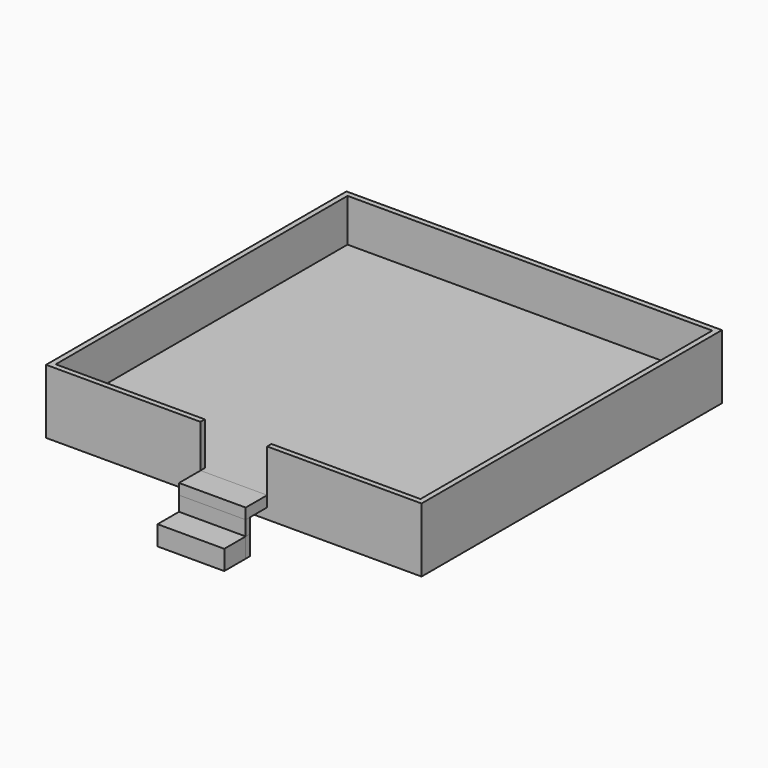
from build123d import *

# Parameters (mm, degrees)
F0_W      = 1778
F0_H      = 1778
F1_DEPTH  = 25.4
F2_W      = 1778
F2_H      = 1778
F2_W_2    = 1727.2
F2_H_2    = 1727.2
F3_DEPTH  = 203.2
F4_W      = 315.869897604
F4_H      = 203.2
F5_DEPTH  = 25.4
F7_DEPTH  = 76.2
F8_W      = 315.869897604
F8_H      = 50.8347044975
F9_DEPTH  = 127
F10_W     = 315.869897604
F10_H     = 69.4447364658
F11_DEPTH = 25.4
F12_W     = 315.869897604
F12_H     = 92.8507968783
F13_DEPTH = 127
F16_DEPTH = 92.8507968783


with BuildPart() as f1:
    # F0 (on Top) → F1 (new body)
    with BuildSketch(Plane.XY):
        Rectangle(F0_W, F0_H)
    extrude(amount=F1_DEPTH)


with BuildPart() as f3:
    # F2 (on face) → F3 (new body)
    with BuildSketch(Plane.XY.offset(25.4)):
        Rectangle(F2_W, F2_H)
        Rectangle(F2_W_2, F2_H_2, mode=Mode.SUBTRACT)
    extrude(amount=F3_DEPTH)

    # F4 (on face) → F5 (cut)
    with BuildSketch(Plane.XZ.offset(889)):
        with Locations((0, 127)):
            Rectangle(F4_W, F4_H)
    extrude(amount=-F5_DEPTH, mode=Mode.SUBTRACT)


with BuildPart() as f1_1:
    add(f1.part)

    # F6: union F3
    add(f3.part)

    # F7 (add): a face of the model
    f7_faces = [f1_1.faces().sort_by_distance(p)[0] for p in [
        (0, 0, 0),
    ]]
    extrude(f7_faces, amount=F7_DEPTH)


with BuildPart() as f9:
    # F8 (on face) → F9 (new body)
    with BuildSketch(Plane.XZ.offset(889)):
        with Locations((0, -0.0173522487)):
            Rectangle(F8_W, F8_H)
    extrude(amount=F9_DEPTH)


with BuildPart() as f11:
    # F10 (on face) → F11 (new body)
    with BuildSketch(Plane.XZ.offset(1016)):
        with Locations((0, -60.1570727304)):
            Rectangle(F10_W, F10_H)
    extrude(amount=-F11_DEPTH)


with BuildPart() as f13:
    # F12 (on face) → F13 (new body)
    with BuildSketch(Plane.XZ.offset(1016)):
        with Locations((0, -141.3048394024)):
            Rectangle(F12_W, F12_H)
    extrude(amount=F13_DEPTH)


with BuildPart() as f16:
    # F16 (new, through all): a face of the model
    f16_faces = [f11.part.faces().sort_by_distance(p)[0] for p in [
        (0, -1003.3, -94.8794409633),
    ]]
    extrude(f16_faces, amount=F16_DEPTH)


solid = Compound([f1_1.part, f9.part, f11.part, f13.part, f16.part])
